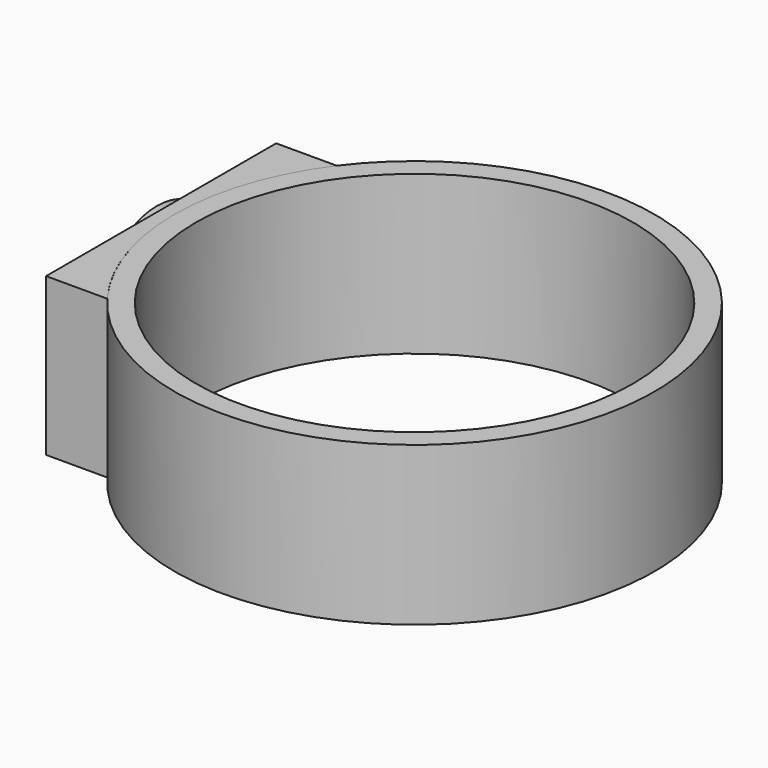
from build123d import *

# Parameters (mm, degrees)
F0_W          = 11.7173120379
F0_H          = 86.0708840191
F3_DEPTH      = 62.484
F3_DEPTH_BACK = 23.114
F4_W          = 156.3523858786
F4_H          = 85.598
F4_R          = 2.5222307947
F5_DEPTH      = 5.08
F6_R          = 26.6100138709


# Not quite as in the source:
# - a feature names something its author has since deleted; it is built from what else it names


with BuildPart() as f1:
    # F0 (on Front) → F1 (revolve)
    with BuildSketch(Plane.XZ):
        with Locations((-22.7350816131, 19.6008179337)):
            Rectangle(F0_W, F0_H)
    revolve(axis=Axis((101.913869381, 0, 19.6008179337), (0, 0, -1)))

    # F2 (on Top) → F3 (join, two sides)
    with BuildSketch(Plane.XY) as f3_sk:
        Polygon((-23.8777473569, 0), (0, 78.1761929393), (-40.9507118165, 78.1761929393), (-40.9507118165, -78.1761929393), (0, -78.1761929393), align=None)
    extrude(amount=F3_DEPTH)
    extrude(f3_sk.sketch, amount=-F3_DEPTH_BACK)

    # F4 (on face) → F5 (cut)
    with BuildSketch(Plane(origin=(-40.9507118165, 0, 0), x_dir=(0, -1, 0), z_dir=(-1, 0, 0))):
        with Locations((0, 19.685)):
            Rectangle(F4_W, F4_H)
        with BuildLine():
            ThreePointArc((-45.8005852997, 15.4996816942), (-31.1457944751, 50.9769783822), (6.1403359286, 60.0954187045))
            ThreePointArc((6.1403359286, 60.0954187045), (28.1936749549, 48.849051517), (43.5657799244, 29.4446982443))
            ThreePointArc((43.5657799244, 29.4446982443), (43.8109995681, 11.2280239142), (37.0950251818, -5.7072364725))
            ThreePointArc((37.0950251818, -5.7072364725), (23.9203018158, -17.178744297), (7.161276415, -22.1086423844))
            ThreePointArc((7.161276415, -22.1086423844), (-16.4091184559, -19.3057274535), (-35.8321219683, -5.6614326371))
            ThreePointArc((-35.8321219683, -5.6614326371), (-42.4741077992, 4.1381986591), (-45.8005852997, 15.4996816942))
        make_face(mode=Mode.SUBTRACT)
        with BuildLine():
            Line((40.1134712131, 27.2007611227), (28.5185842412, 21.4439421826))
            Line((28.5185842412, 21.4439421826), (28.5185842412, 17.7521709857))
            Line((28.5185842412, 17.7521709857), (-25.6030233871, 17.7521709857))
            ThreePointArc((-25.6030233871, 17.7521709857), (-16.3053602602, 2.8665512096), (0, -3.6267871095))
            Line((0, -3.6267871095), (0, -7.4742618075))
            ThreePointArc((0, -7.4742618075), (-3.0208305793, -7.2095008507), (-6.0036519209, -6.6633391553))
            Line((-6.0036519209, -6.6633391553), (-10.9303286299, -16.9180645665))
            ThreePointArc((-10.9303286299, -16.9180645665), (27.850277377, -10.1984693401), (40.1134712131, 27.2007611227))
        make_face()
        with Locations((-14.9526894093, 12.6375420892)):
            Circle(F4_R, mode=Mode.SUBTRACT)
        with BuildLine():
            Line((-30.2748965285, 18.925355512), (-30.2748965285, 22.6689743163))
            Line((-30.2748965285, 22.6689743163), (23.6969497055, 22.6689743163))
            ThreePointArc((23.6969497055, 22.6689743163), (14.8585733056, 36.2512107395), (0, 42.7178051265))
            Line((0, 42.7178051265), (0, 46.5652798245))
            ThreePointArc((0, 46.5652798245), (2.7362509253, 46.2128562393), (5.4325754525, 45.6288138147))
            Line((5.4325754525, 45.6288138147), (10.3592521615, 55.8835392259))
            ThreePointArc((10.3592521615, 55.8835392259), (-28.2973985554, 49.8617154144), (-41.8697835003, 13.1685365719))
            Line((-41.8697835003, 13.1685365719), (-30.2748965285, 18.925355512))
        make_face()
        with Locations((10.5805564672, 29.0767555067)):
            Circle(F4_R, mode=Mode.SUBTRACT)
        with BuildLine():
            ThreePointArc((-23.5536272178, -10.4727910391), (-19.567339601, -12.673386574), (-15.5009556321, -14.7221986906))
            Line((-15.5009556321, -14.7221986906), (-10.8854688828, -5.1152055697))
            ThreePointArc((-10.8854688828, -5.1152055697), (-13.7327556617, -3.7930202048), (-16.4386400958, -2.2013526611))
            Line((-16.4386400958, -2.2013526611), (-23.5536272178, -10.4727910391))
        make_face()
        with BuildLine():
            ThreePointArc((-26.5336921008, 8.3536629544), (-27.9587005711, 11.0330778371), (-29.1266296715, 13.8341231545))
            Line((-29.1266296715, 13.8341231545), (-39.6148164121, 8.6267768283))
            ThreePointArc((-39.6148164121, 8.6267768283), (-37.8198393057, 5.3233394517), (-35.7862055506, 2.1612238524))
            Line((-35.7862055506, 2.1612238524), (-26.5336921008, 8.3536629544))
        make_face()
        with BuildLine():
            ThreePointArc((22.037269041, 49.3868926394), (18.5082065055, 51.5635703889), (14.8724930701, 53.5570086801))
            Line((14.8724930701, 53.5570086801), (10.2570063209, 43.9500155592))
            ThreePointArc((10.2570063209, 43.9500155592), (12.731329703, 42.7351985505), (15.0933792595, 41.3143613127))
            Line((15.0933792595, 41.3143613127), (22.037269041, 49.3868926394))
        make_face()
        with BuildLine():
            ThreePointArc((24.8030604194, 31.2912532728), (26.1088071334, 28.9630296891), (27.2183651143, 26.5351745401))
            Line((27.2183651143, 26.5351745401), (37.7065518548, 31.7425208664))
            ThreePointArc((37.7065518548, 31.7425208664), (36.0872429679, 34.7420367782), (34.1578114173, 37.5521170028))
            Line((34.1578114173, 37.5521170028), (24.8030604194, 31.2912532728))
        make_face()
        with BuildLine():
            ThreePointArc((-20.4539452974, 0.9064794757), (-22.0908205991, 2.5015221962), (-23.6111177136, 4.2080446007))
            Line((-23.6111177136, 4.2080446007), (-32.9658687115, -2.0528191293))
            ThreePointArc((-32.9658687115, -2.0528191293), (-30.4877258305, -4.9425156474), (-27.3978350789, -7.166051851))
            Line((-27.3978350789, -7.166051851), (-20.4539452974, 0.9064794757))
        make_face()
        with BuildLine():
            ThreePointArc((19.0953313845, 38.1919350162), (20.4937445485, 36.8328627443), (21.8078204864, 35.3920847438))
            Line((21.8078204864, 35.3920847438), (31.0603339362, 41.5845238458))
            ThreePointArc((31.0603339362, 41.5845238458), (28.7909533219, 44.1786559607), (26.2103185065, 46.4633733942))
            Line((26.2103185065, 46.4633733942), (19.0953313845, 38.1919350162))
        make_face()
    extrude(amount=-F5_DEPTH, mode=Mode.SUBTRACT)

    # F6
    f6_edges = [f1.edges().sort_by_distance(p)[0] for p in [
        (-38.410712, -43.56578, 29.444698),
    ]]
    fillet(f6_edges, radius=F6_R)


solid = f1.part
